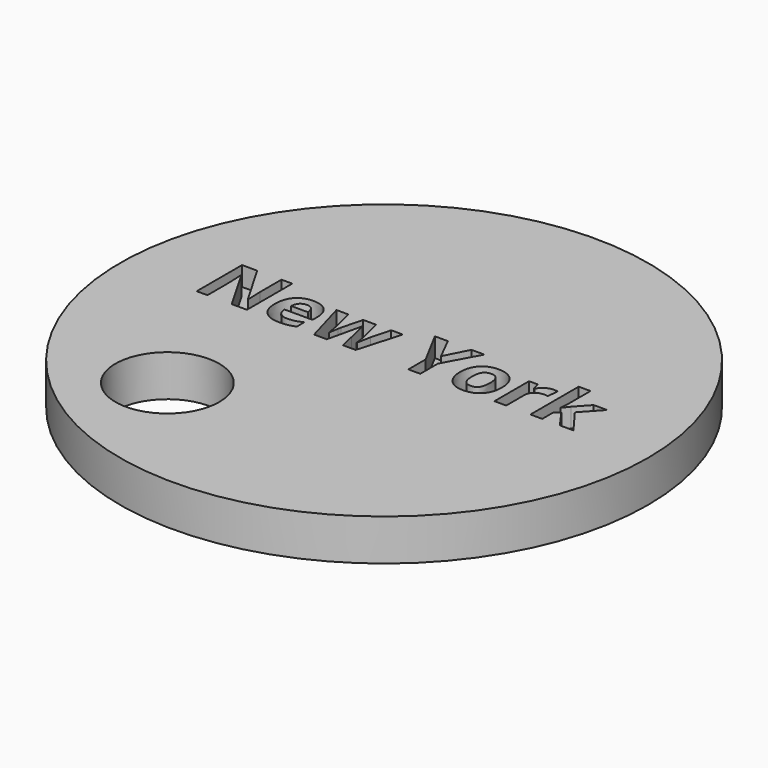
from build123d import *

# Parameters (mm, degrees)
F0_R         = 13.7
F1_DEPTH     = 2.15
F2_R         = 2.6941000827
F3_DEPTH     = 25
F4_TEXT_SIZE = 4.1191699155
F5_DEPTH     = 1


# Not quite as in the source:
# - Text() gives the source's letters only with a copy of the font that has no kerning and outlines rounded to 1/6400 em; it was checked with that copy


with BuildPart() as f1:
    # F0 (on Top) → F1 (new body)
    with BuildSketch(Plane.XY):
        Circle(F0_R)
    extrude(amount=F1_DEPTH)

    # F2 (on face) → F3 (cut)
    with BuildSketch(Plane.XY.offset(2.15)):
        with Locations((-5.6303618476, -7.0227142423)):
            Circle(F2_R)
    extrude(amount=-F3_DEPTH, mode=Mode.SUBTRACT)

    # F4 (on face) → F5 (cut)
    with BuildSketch(Plane.XY.offset(2.15)):
        with Locations((-10.0958280148, 0)):
            Text('New York', F4_TEXT_SIZE, font='Open Sans', font_style=FontStyle.BOLD, text_align=(TextAlign.LEFT, TextAlign.BOTTOM))
    extrude(amount=-F5_DEPTH, mode=Mode.SUBTRACT)


solid = f1.part
